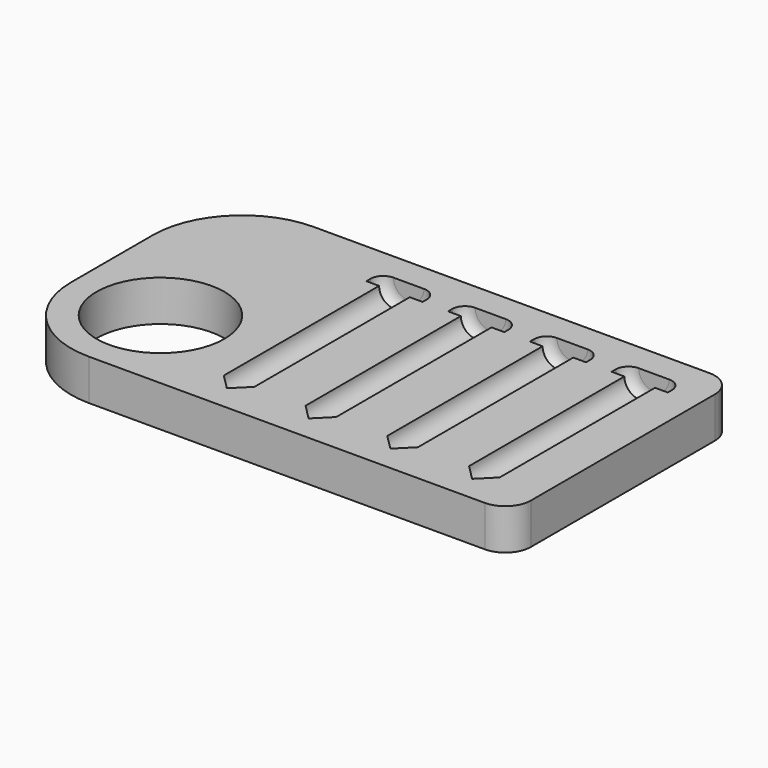
from build123d import *

# Parameters (mm, degrees)
F0_R         = 12.5
F1_DEPTH     = 8
F7_TEXT_SIZE = 5.5555555556
F8_DEPTH     = 1


# Not quite as in the source:
# - Text() gives the source's letters only with a copy of the font that has no kerning and outlines rounded to 1/6400 em; it was checked with that copy


with BuildPart() as f1:
    # F0 (on Top) → F1 (new body)
    with BuildSketch(Plane.XY):
        with BuildLine():
            ThreePointArc((0, 17.5), (5.1256313292, 5.1256313292), (17.5, 0))
            Line((17.5, 0), (95, 0))
            ThreePointArc((95, 0), (98.5355339059, 1.4644660941), (100, 5))
            Line((100, 5), (100, 50))
            ThreePointArc((100, 50), (98.5355339059, 53.5355339059), (95, 55))
            Line((95, 55), (17.5, 55))
            ThreePointArc((17.5, 55), (5.1256313292, 49.8743686708), (0, 37.5))
            Line((0, 37.5), (0, 17.5))
        make_face()
        with Locations((17.5, 17.5)):
            Circle(F0_R, mode=Mode.SUBTRACT)
    extrude(amount=F1_DEPTH)

    # F2 (on face) → F3 (revolve, cut)
    with BuildSketch(Plane.XY.offset(8)):
        with BuildLine():
            Line((40.5, 46), (40.5, 5))
            Line((40.5, 5), (43.5, 8))
            Line((43.5, 8), (43.5, 46))
            Line((43.5, 46), (46, 46))
            Line((46, 46), (46, 47))
            ThreePointArc((46, 47), (45.267766953, 48.767766953), (43.5, 49.5))
            Line((43.5, 49.5), (40.5, 49.5))
            Line((40.5, 49.5), (40.5, 46))
        make_face()
    revolve(axis=Axis((40.5, 25.5, 8), (0, 1, 0)), mode=Mode.SUBTRACT)

    # F2 (on face) → F4 (revolve, cut)
    with BuildSketch(Plane.XY.offset(8)):
        with BuildLine():
            Line((56.5, 46), (56.5, 5))
            Line((56.5, 5), (59.5, 8))
            Line((59.5, 8), (59.5, 46))
            Line((59.5, 46), (62, 46))
            Line((62, 46), (62, 47))
            ThreePointArc((62, 47), (61.267766953, 48.767766953), (59.5, 49.5))
            Line((59.5, 49.5), (56.5, 49.5))
            Line((56.5, 49.5), (56.5, 46))
        make_face()
    revolve(axis=Axis((56.5, 25.5, 8), (0, 1, 0)), mode=Mode.SUBTRACT)

    # F2 (on face) → F5 (revolve, cut)
    with BuildSketch(Plane.XY.offset(8)):
        with BuildLine():
            Line((72.5, 46), (72.5, 5))
            Line((72.5, 5), (75.5, 8))
            Line((75.5, 8), (75.5, 46))
            Line((75.5, 46), (78, 46))
            Line((78, 46), (78, 47))
            ThreePointArc((78, 47), (77.267766953, 48.767766953), (75.5, 49.5))
            Line((75.5, 49.5), (72.5, 49.5))
            Line((72.5, 49.5), (72.5, 46))
        make_face()
    revolve(axis=Axis((72.5, 25.5, 8), (0, 1, 0)), mode=Mode.SUBTRACT)

    # F2 (on face) → F6 (revolve, cut)
    with BuildSketch(Plane.XY.offset(8)):
        with BuildLine():
            Line((88.5, 46), (88.5, 5))
            Line((88.5, 5), (91.5, 8))
            Line((91.5, 8), (91.5, 46))
            Line((91.5, 46), (94, 46))
            Line((94, 46), (94, 47))
            ThreePointArc((94, 47), (93.267766953, 48.767766953), (91.5, 49.5))
            Line((91.5, 49.5), (88.5, 49.5))
            Line((88.5, 49.5), (88.5, 46))
        make_face()
    revolve(axis=Axis((88.5, 25.5, 8), (0, 1, 0)), mode=Mode.SUBTRACT)

    # F7 (on face) → F8 (cut)
    with BuildSketch(Plane(origin=(0, 0, 0), x_dir=(1, 0, 0), z_dir=(0, 0, -1))):
        with Locations((30, -9)):
            Text('995', F7_TEXT_SIZE, font='Open Sans', text_align=(TextAlign.LEFT, TextAlign.BOTTOM))
    extrude(amount=-F8_DEPTH, mode=Mode.SUBTRACT)


solid = f1.part
